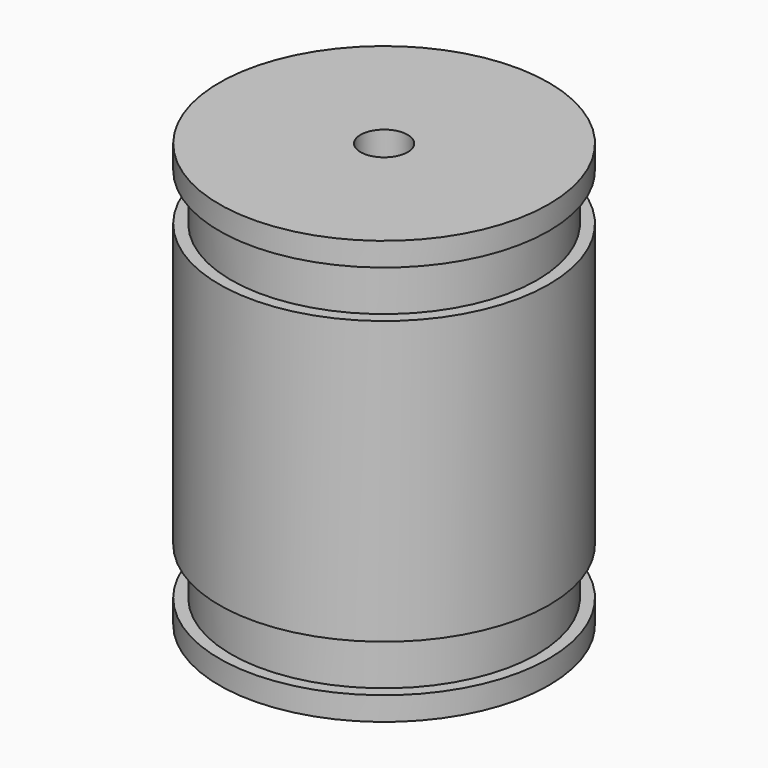
from build123d import *

# Parameters (mm, degrees)
F4_R     = 3.175
F5_DEPTH = 57.151
F6_R     = 1.3081


with BuildPart() as f1:
    # F0 (on Front) → F1 (revolve)
    with BuildSketch(Plane.XZ):
        Polygon((22.225, 0), (0, 0), (0, -12.7), (10.16, -12.7), (10.16, -57.15), (22.225, -57.15), (22.225, -53.975), (20.6375, -53.975), (20.6375, -47.625), (22.225, -47.625), (22.225, -9.525), (20.6375, -9.525), (20.6375, -3.175), (22.225, -3.175), align=None)
    revolve(axis=Axis((0, 0, -6.35), (0, 0, 1)))

    # F4 (on face) → F5 (cut, through all)
    with BuildSketch(Plane.XY):
        Circle(F4_R)
    extrude(amount=-F5_DEPTH, mode=Mode.SUBTRACT)


with BuildPart() as f3:
    # F2 (on Right) → F3 (revolve)
    with BuildSketch(Plane.YZ):
        Polygon((9.906, -28.575), (0, -28.575), (0, -53.975), (9.906, -53.975), (9.906, -34.3662), (8.0518, -34.3662), (8.0518, -31.75), (9.906, -31.75), align=None)
    revolve(axis=Axis((0, 0, -41.275), (0, 0, -1)))


with BuildPart() as f7:
    # F6 (on Right) → F7 (revolve)
    with BuildSketch(Plane.YZ):
        with Locations((9.350375, -33.0581)):
            Circle(F6_R)
    revolve(axis=Axis((0, 0, -30.0969633236), (0, 0, 1)))


solid = Compound([f1.part, f3.part, f7.part])
